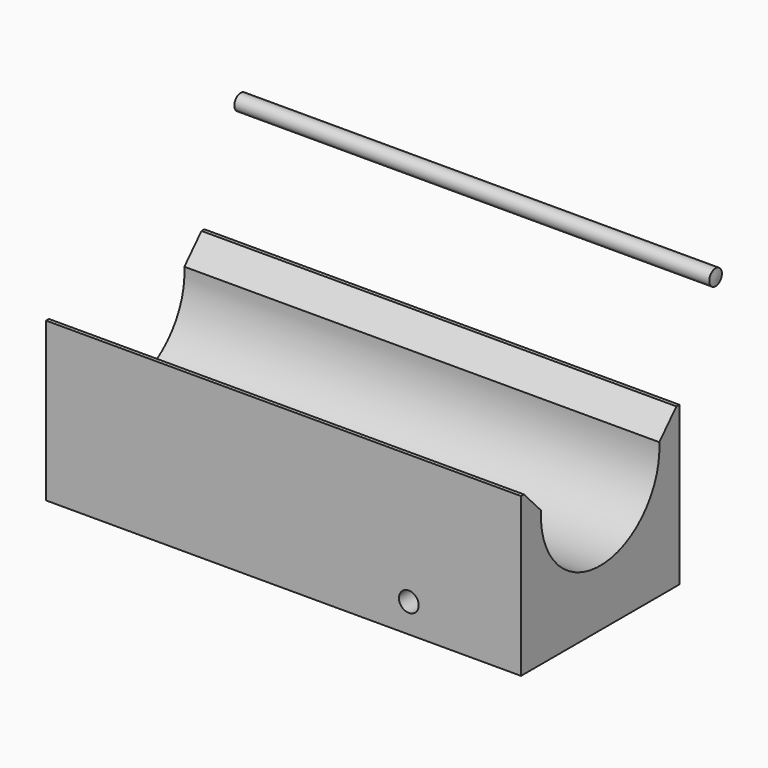
from build123d import *

# Parameters (mm, degrees)
F0_W        = 76.2
F0_H        = 25.4
F1_DEPTH    = 15.875
F2_R        = 11.8831121617
F3_DEPTH    = 76.2
F4_T1_DEPTH = 98.1986886944
F5_R        = 1.5875
F6_DEPTH    = 76.2


# Not quite as in the source:
# - a fillet or chamfer that OpenCascade refuses, or shapes differently, is made with other operations: its cross-section is extruded or revolved along the edge and cut away or added


with BuildPart() as f1:
    # F0 (on Front) → F1 (new body, symmetric)
    with BuildSketch(Plane.XZ):
        with Locations((-6.1091389507, 16.743282738)):
            Rectangle(F0_W, F0_H)
    extrude(amount=F1_DEPTH, both=True)

    # F2 (on Right) → F3 (cut, symmetric)
    with BuildSketch(Plane.YZ):
        with Locations((0, 25.0277593732)):
            Circle(F2_R)
    extrude(amount=F3_DEPTH, both=True, mode=Mode.SUBTRACT)

    # F4: chamfer of 5.08 on 2 edges, made by hand

    # F4_s2 → F4_t1 (cut)
    with BuildSketch(Plane.YZ.offset(-55.2084832979)):
        with BuildLine():
            Line((15.4295351274, 29.5914768875), (11.7199033612, 25.6372630168))
            Line((11.7199033612, 25.6372630168), (11.6185101073, 25.6307847395))
            ThreePointArc((11.6185101073, 25.6307847395), (11.5042711471, 27.5685809315), (10.937968324, 29.4055302395))
            Line((10.937968324, 29.4055302395), (11.0322938713, 29.544882738))
            ThreePointArc((11.0322938713, 29.544882738), (13.2309144993, 29.544882738), (15.4295351274, 29.6930768875))
            Line((15.4295351274, 29.6930768875), (15.4295351274, 29.5914768875))
        make_face()
        with BuildLine():
            Line((-15.4295351274, 29.5914768875), (-11.7199033612, 25.6372630168))
            Line((-11.7199033612, 25.6372630168), (-11.6185101073, 25.6307847395))
            ThreePointArc((-11.6185101073, 25.6307847395), (-11.5042711471, 27.5685809315), (-10.937968324, 29.4055302395))
            Line((-10.937968324, 29.4055302395), (-11.0322938713, 29.544882738))
            ThreePointArc((-11.0322938713, 29.544882738), (-13.2309144993, 29.544882738), (-15.4295351274, 29.6930768875))
            Line((-15.4295351274, 29.6930768875), (-15.4295351274, 29.5914768875))
        make_face()
    extrude(amount=F4_T1_DEPTH, mode=Mode.SUBTRACT)

    # F5 (on Front) → F6 (cut, symmetric)
    with BuildSketch(Plane.XZ):
        with Locations((13.9918969944, 8.6710350588)):
            Circle(F5_R)
    extrude(amount=F6_DEPTH, both=True, mode=Mode.SUBTRACT)


with BuildPart() as f8:
    # F7 (on Front) → F8 (revolve)
    with BuildSketch(Plane.XZ):
        Polygon((50.6395318134, 59.9220860207), (50.5097051469, 61.1920860207), (-25.6902948531, 61.1920860207), (-25.6902948531, 59.9220860207), align=None)
    revolve(axis=Axis((12.4746184802, 0, 59.9220860207), (1, 0, 0)))


solid = Compound([f1.part, f8.part])
